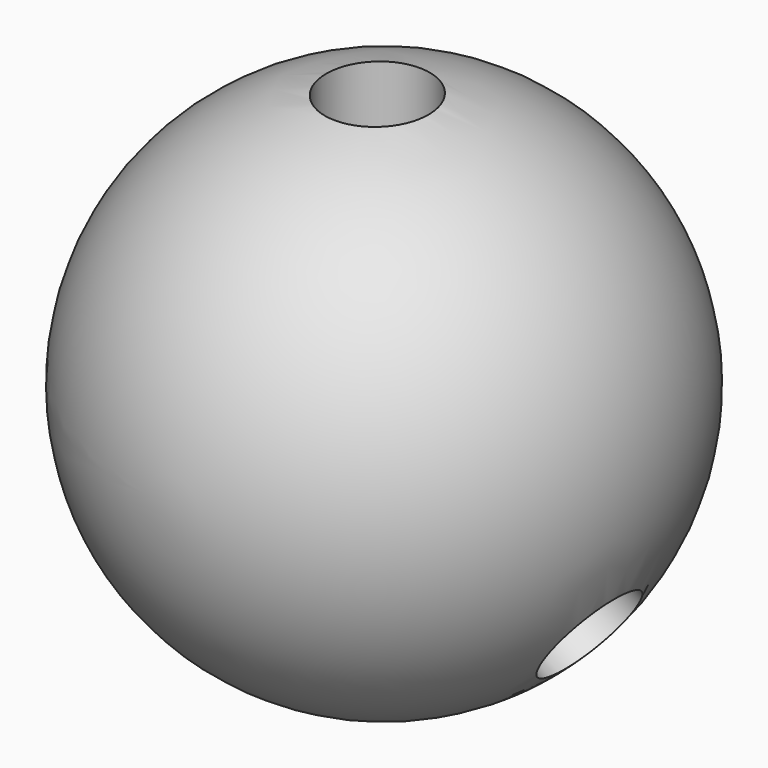
from build123d import *

# Parameters (mm, degrees)
F4_R          = 3.175
F5_DEPTH      = 38.1
F6_ANGLE      = 124.9
F8_ANGLE      = -124.9
F9_TEXT_SIZE  = 2.0345537147
F10_DEPTH     = 7.112
F12_TEXT_SIZE = 4.0888850991
F13_DEPTH     = 7.6708


# Not quite as in the source:
# - Text() gives the source's letters only with a copy of the font that has no kerning and outlines rounded to 1/6400 em; it was checked with that copy


with BuildPart() as f1:
    # F0 (on Top) → F1 (revolve)
    with BuildSketch(Plane.XY):
        with BuildLine():
            Line((0, -15.3701132685), (0, 16.3798867315))
            ThreePointArc((0, 16.3798867315), (-15.875, 0.5048867315), (0, -15.3701132685))
        make_face()
    revolve(axis=Axis((0, 0.5048867315, 0), (0, -1, 0)))

    # F9 (on offset) → F10 (cut)
    with BuildSketch(Plane(origin=(15.6238932354, 0, -10.8993788891), x_dir=(0, 1, 0), z_dir=(0.8201518759, 0, -0.5721458734))):
        with Locations((-2.2461470217, -5.5665364489)):
            Text('124.9', F9_TEXT_SIZE, font='Open Sans', text_align=(TextAlign.LEFT, TextAlign.BOTTOM))
    extrude(amount=-F10_DEPTH, mode=Mode.SUBTRACT)

    # F12 (on offset) → F13 (cut)
    with BuildSketch(Plane(origin=(-17.8782920836, 0, -6.5779306909), x_dir=(0, -1, 0), z_dir=(-0.9384930228, 0, -0.345298199))):
        with Locations((-3.3571780659, 4.2501757853)):
            Text('110.2', F12_TEXT_SIZE, font='Open Sans', text_align=(TextAlign.LEFT, TextAlign.BOTTOM))
    extrude(amount=-F13_DEPTH, mode=Mode.SUBTRACT)


with BuildPart() as f5:
    # F4 (on offset) → F5 (new body)
    with BuildSketch(Plane.XY.offset(6.35)):
        Circle(F4_R)
    extrude(amount=F5_DEPTH)


with BuildPart() as f6_1:
    # F6: copy of F5
    add(f5.part.rotate(Axis((0, 26.7314519733, 0), (0, 1, 0)), F6_ANGLE))


with BuildPart() as f8_1:
    # F8: copy of F6_1
    add(f6_1.part.rotate(Axis((0, 0.5048867315, 0), (0, -1, 0)), F8_ANGLE))


with BuildPart() as f1_1:
    add(f1.part)

    # F14: cut F6_1, F5, F8_1
    add(f6_1.part, mode=Mode.SUBTRACT)
    add(f5.part, mode=Mode.SUBTRACT)
    add(f8_1.part, mode=Mode.SUBTRACT)


solid = f1_1.part
